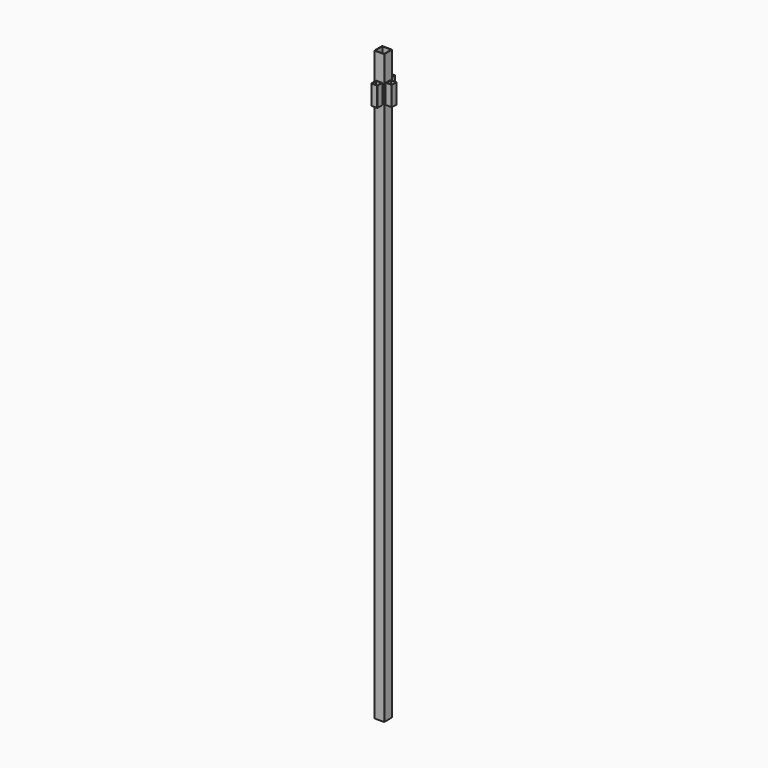
from build123d import *

# Parameters (mm, degrees)
F0_W            = 45.8
F0_H            = 45.8
F1_DEPTH        = 3000
F2_W            = 31.75
F2_H            = 100
F3_DEPTH        = 31.75
F3_COPIES_COUNT = 3
F3_COPIES_ANGLE = 180
F4_R            = 2.5
F5_W            = 26.75
F5_H            = 26.75
F6_DEPTH        = 100
F6_COPIES_COUNT = 3
F6_COPIES_ANGLE = 180


# Not quite as in the source:
# - a pattern or mirror of a feature is missing from the dataset's text; its kind, count and spacing are read off the source's solid


with BuildPart() as f1:
    # F0 (on Top) → F1 (new body)
    with BuildSketch(Plane.XY):
        with BuildLine():
            ThreePointArc((25.4, 22.9), (24.667766953, 24.667766953), (22.9, 25.4))
            Line((22.9, 25.4), (-22.9, 25.4))
            ThreePointArc((-22.9, 25.4), (-24.667766953, 24.667766953), (-25.4, 22.9))
            Line((-25.4, 22.9), (-25.4, -22.9))
            ThreePointArc((-25.4, -22.9), (-24.667766953, -24.667766953), (-22.9, -25.4))
            Line((-22.9, -25.4), (22.9, -25.4))
            ThreePointArc((22.9, -25.4), (24.667766953, -24.667766953), (25.4, -22.9))
            Line((25.4, -22.9), (25.4, 22.9))
        make_face()
        Rectangle(F0_W, F0_H, mode=Mode.SUBTRACT)
    extrude(amount=F1_DEPTH)

    # F2 (on face) → F3 (join)
    with BuildSketch(Plane.XZ.offset(25.4)):
        with Locations((0, 2818.25)):
            Rectangle(F2_W, F2_H)
    f3 = extrude(amount=F3_DEPTH)

    # F3_copies: F3 ×3 about axis
    f3_copies_axis = Axis((0, 0, 0), (0, 0, 1))
    for i in range(1, F3_COPIES_COUNT):
        add(f3.rotate(f3_copies_axis, i * F3_COPIES_ANGLE / (F3_COPIES_COUNT - 1)))

    # F4
    f4_edges = [f1.edges().sort_by_distance(p)[0] for p in [
        (-15.875, -57.15, 2818.25),
        (15.875, -57.15, 2818.25),
        (57.15, -15.875, 2818.25),
        (57.15, 15.875, 2818.25),
        (15.875, 57.15, 2818.25),
        (-15.875, 57.15, 2818.25),
    ]]
    fillet(f4_edges, radius=F4_R)

    # F5 (on face) → F6 (cut, through all)
    with BuildSketch(Plane.XY.offset(2868.25)):
        with Locations((0, -41.275)):
            Rectangle(F5_W, F5_H)
    f6 = extrude(amount=-F6_DEPTH, mode=Mode.SUBTRACT)

    # F6_copies: F6 ×3 about axis
    f6_copies_axis = Axis((0, 0, 0), (0, 0, 1))
    for i in range(1, F6_COPIES_COUNT):
        add(f6.rotate(f6_copies_axis, i * F6_COPIES_ANGLE / (F6_COPIES_COUNT - 1)), mode=Mode.SUBTRACT)


solid = f1.part
